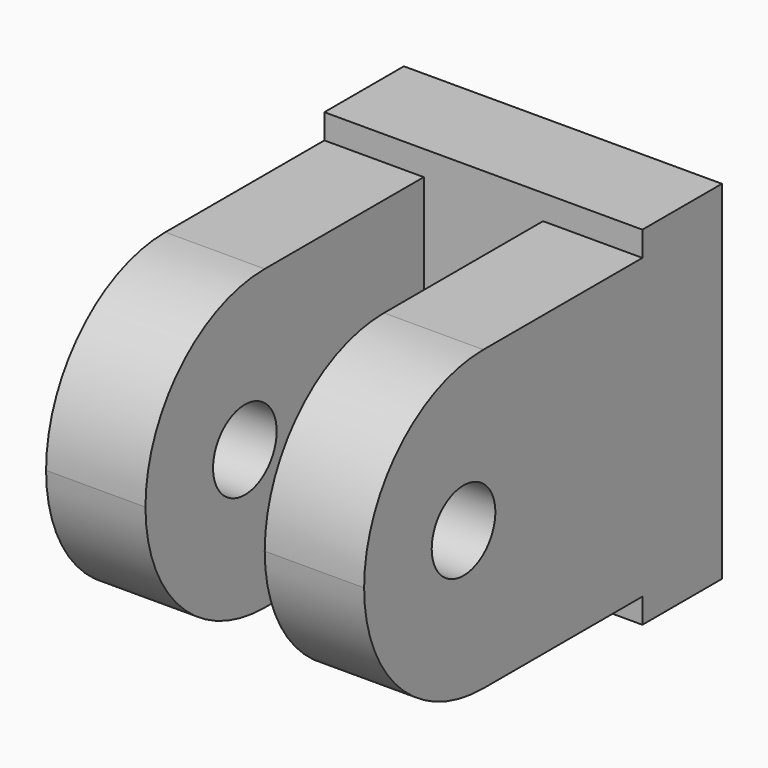
from build123d import *

# Parameters (mm, degrees)
F0_W      = 32
F0_H      = 35
F1_DEPTH  = 10
F2_W      = 10
F2_H      = 30
F3_DEPTH  = 35
F4_R      = 4
F5_DEPTH  = 10.001
F6_R      = 4
F7_DEPTH  = 10.001
F8_R      = 14.99999
F9_R      = 2
F10_DEPTH = 10.001


# Not quite as in the source:
# - a fillet or chamfer is up to 0.001 mm smaller than in the source, because OpenCascade refuses the exact size


with BuildPart() as f1:
    # F0 (on Front) → F1 (new body)
    with BuildSketch(Plane.XZ):
        Rectangle(F0_W, F0_H)
    extrude(amount=F1_DEPTH)

    # F2 (on face) → F3 (join)
    with BuildSketch(Plane.XZ.offset(10)):
        with Locations((-11, 0)):
            Rectangle(F2_W, F2_H)
        with Locations((11, 0)):
            Rectangle(F2_W, F2_H)
    extrude(amount=F3_DEPTH)

    # F4 (on face) → F5 (cut, through all)
    with BuildSketch(Plane.YZ.offset(-6)):
        with Locations((-32.5, 0)):
            Circle(F4_R)
    extrude(amount=-F5_DEPTH, mode=Mode.SUBTRACT)

    # F6 (on face) → F7 (cut, through all)
    with BuildSketch(Plane(origin=(6, 0, 0), x_dir=(0, -1, 0), z_dir=(-1, 0, 0))):
        with Locations((32.5, 0)):
            Circle(F6_R)
    extrude(amount=-F7_DEPTH, mode=Mode.SUBTRACT)

    # F8 (radius 15 in the source; OpenCascade refuses exactly that, so slightly less here)
    f8_edges = [f1.edges().sort_by_distance(p)[0] for p in [
        (-11, -45, -15),
        (11, -45, -15),
        (-11, -45, 15),
        (11, -45, 15),
    ]]
    fillet(f8_edges, radius=F8_R)

    # F9 (on face) → F10 (cut, through all)
    with BuildSketch(Plane.XZ.offset(10)):
        with Locations((0, 5)):
            Circle(F9_R)
        with Locations((0, -5)):
            Circle(F9_R)
    extrude(amount=-F10_DEPTH, mode=Mode.SUBTRACT)


solid = f1.part
